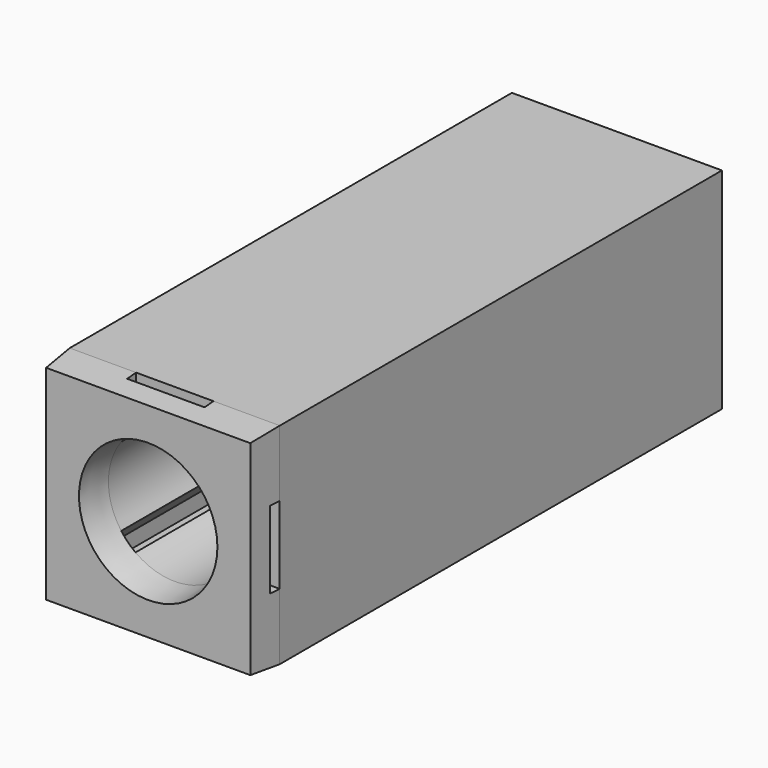
from build123d import *

# Parameters (mm, degrees)
F0_W            = 19
F0_H            = 19
F0_W_2          = 17
F0_H_2          = 17
F1_DEPTH        = 50
F2_W            = 16.7
F2_H            = 16.7
F2_R            = 6
F3_DEPTH        = 15
F4_W            = 19
F4_H            = 19
F4_R            = 6
F5_DEPTH        = 3
F5_TAPER        = 5
F6_W            = 7
F6_H            = 1
F7_DEPTH        = 1.15
F7_COPIES_COUNT = 4
F8_SIZE         = 2
F10_DEPTH       = 15


# Not quite as in the source:
# - a pattern or mirror of a feature is missing from the dataset's text; its kind, count and spacing are read off the source's solid


with BuildPart() as f1:
    # F0 (on Front) → F1 (new body)
    with BuildSketch(Plane.XZ):
        Rectangle(F0_W, F0_H)
        Rectangle(F0_W_2, F0_H_2, mode=Mode.SUBTRACT)
    extrude(amount=-F1_DEPTH)


with BuildPart() as f3:
    # F2 (on face) → F3 (new body)
    with BuildSketch(Plane.XZ):
        Rectangle(F2_W, F2_H)
        Circle(F2_R, mode=Mode.SUBTRACT)
    extrude(amount=-F3_DEPTH)

    # F4 (on face) → F5 (join)
    with BuildSketch(Plane.XZ):
        Rectangle(F4_W, F4_H)
        Circle(F4_R, mode=Mode.SUBTRACT)
    extrude(amount=F5_DEPTH, taper=F5_TAPER)

    # F6 (on face) → F7 (cut)
    with BuildSketch(Plane.XY.offset(9.5)):
        with Locations((0, -0.5)):
            Rectangle(F6_W, F6_H)
        with Locations((0, 0.5)):
            Rectangle(F6_W, F6_H)
    f7 = extrude(amount=-F7_DEPTH, mode=Mode.SUBTRACT)

    # F7_copies: F7 ×4 about axis
    f7_copies_axis = Axis((0, 0, 0), (0, 1, 0))
    for i in range(1, F7_COPIES_COUNT):
        add(f7.rotate(f7_copies_axis, i * 360 / F7_COPIES_COUNT), mode=Mode.SUBTRACT)

    # F8
    f8_edges = [f3.edges().sort_by_distance(p)[0] for p in [
        (8.35, 7.5, 8.35),
        (8.35, 7.5, -8.35),
        (-8.35, 7.5, -8.35),
        (-8.35, 7.5, 8.35),
    ]]
    chamfer(f8_edges, length=F8_SIZE)

    # F9 (on face) → F10 (cut, through all)
    with BuildSketch(Plane(origin=(0, 15, 0), x_dir=(-1, 0, 0), z_dir=(0, 1, 0))):
        with BuildLine():
            Line((7.9964466094, 6.7035533906), (6.7035533906, 7.9964466094))
            Line((6.7035533906, 7.9964466094), (3.5466556766, 4.8395488954))
            ThreePointArc((3.5466556766, 4.8395488954), (4.2426406871, 4.2426406871), (4.8395488954, 3.5466556766))
            Line((4.8395488954, 3.5466556766), (7.9964466094, 6.7035533906))
        make_face()
        Polygon((12.7629971477, 14.0558903665), (6.7035533906, 7.9964466094), (7.9964466094, 6.7035533906), (13.9659964202, 12.6731032014), align=None)
        with BuildLine():
            ThreePointArc((4.8395488954, 3.5466556766), (4.2426406871, 4.2426406871), (3.5466556766, 4.8395488954))
            Line((3.5466556766, 4.8395488954), (-4.8395488954, -3.5466556766))
            ThreePointArc((-4.8395488954, -3.5466556766), (-4.2426406871, -4.2426406871), (-3.5466556766, -4.8395488954))
            Line((-3.5466556766, -4.8395488954), (4.8395488954, 3.5466556766))
        make_face()
        with BuildLine():
            ThreePointArc((-3.5466556766, -4.8395488954), (-4.2426406871, -4.2426406871), (-4.8395488954, -3.5466556766))
            Line((-4.8395488954, -3.5466556766), (-7.9964466094, -6.7035533906))
            Line((-7.9964466094, -6.7035533906), (-6.7035533906, -7.9964466094))
            Line((-6.7035533906, -7.9964466094), (-3.5466556766, -4.8395488954))
        make_face()
        Polygon((-6.7035533906, -7.9964466094), (-7.9964466094, -6.7035533906), (-11.6992480187, -10.4063547999), (-10.4063547999, -11.6992480187), align=None)
    f10 = extrude(amount=-F10_DEPTH, mode=Mode.SUBTRACT)

    # F10_copies: F10 across plane
    add(f10.mirror(Plane(origin=(0, 0, 0), x_dir=(0, 0, 1), z_dir=(1, 0, 0))), mode=Mode.SUBTRACT)


solid = Compound([f1.part, f3.part])
